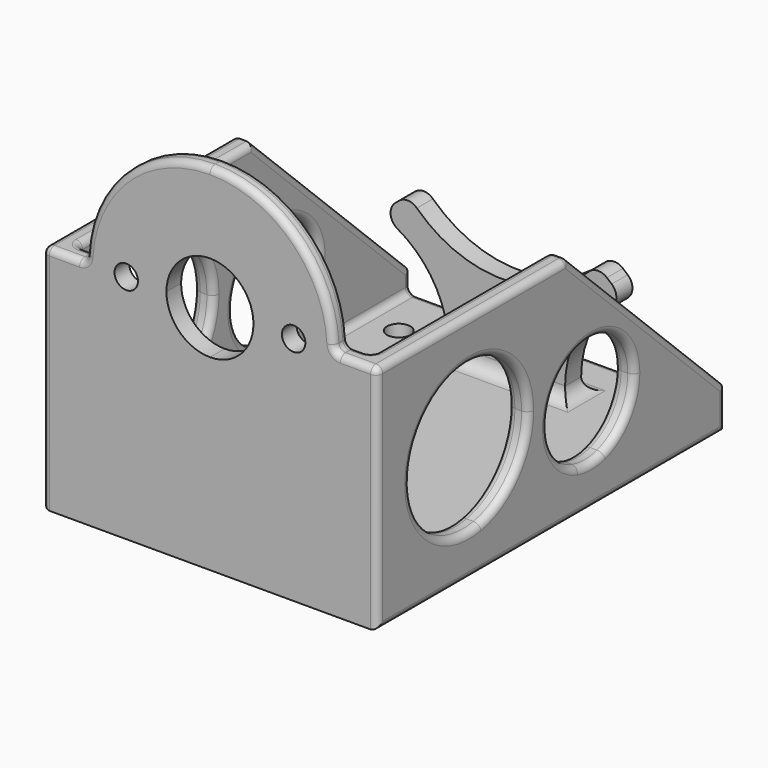
from build123d import *

# Parameters (mm, degrees)
F0_W      = 50
F0_H      = 65
F1_DEPTH  = 53
F2_W      = 44
F2_H      = 64
F3_DEPTH  = 50
F5_DEPTH  = 50.8
F6_R      = 1.75
F7_DEPTH  = 46.482
F9_DEPTH  = 51.054
F10_R     = 1
F12_DEPTH = 25.4
F14_DEPTH = 31.5
F16_DEPTH = 25.4
F17_R     = 2


with BuildPart() as f1:
    # F0 (on Top) → F1 (new body)
    with BuildSketch(Plane.XY):
        Rectangle(F0_W, F0_H)
    extrude(amount=F1_DEPTH)

    # F2 (on face) → F3 (cut)
    with BuildSketch(Plane.XY.offset(53)):
        with Locations((0, 2.2385166958)):
            Rectangle(F2_W, F2_H)
    extrude(amount=-F3_DEPTH, mode=Mode.SUBTRACT)

    # F4 (on face) → F5 (cut)
    with BuildSketch(Plane.YZ.offset(25)):
        Polygon((32.5, 53), (-16.1271169782, 53), (32.5, 6.0290149413), align=None)
    extrude(amount=-F5_DEPTH, mode=Mode.SUBTRACT)

    # F6 (on face) → F7 (cut)
    with BuildSketch(Plane.XZ.offset(32.5)):
        with Locations((-12.5, 34.5)):
            Circle(F6_R)
        with BuildLine():
            ThreePointArc((14.25, 34.5), (12.5, 36.25), (10.75, 34.5))
            ThreePointArc((10.75, 34.5), (12.5, 32.75), (14.25, 34.5))
        make_face()
        with BuildLine():
            Line((-6.5, 34.5), (0, 34.5))
            Line((0, 34.5), (6.5, 34.5))
            ThreePointArc((6.5, 34.5), (0, 41), (-6.5, 34.5))
        make_face()
        with BuildLine():
            Line((0, 34.5), (0, 28))
            ThreePointArc((0, 28), (4.5961940777, 29.9038059223), (6.5, 34.5))
            Line((6.5, 34.5), (0, 34.5))
        make_face()
        with BuildLine():
            ThreePointArc((-6.5, 34.5), (-4.5961940777, 29.9038059223), (0, 28))
            Line((0, 28), (0, 34.5))
            Line((0, 34.5), (-6.5, 34.5))
        make_face()
        with BuildLine():
            Line((-25, 34.5), (-18.5, 34.5))
            ThreePointArc((-18.5, 34.5), (-13.0814754005, 47.5814755034), (1.455e-07, 53))
            Line((1.455e-07, 53), (-25, 53))
            Line((-25, 53), (-25, 34.5))
        make_face()
        with BuildLine():
            Line((18.4999672276, 34.5348220845), (25, 34.5348220845))
            Line((25, 34.5348220845), (25, 53))
            Line((25, 53), (1.455e-07, 53))
            ThreePointArc((1.455e-07, 53), (13.0691582386, 47.5937810787), (18.4999672276, 34.5348220845))
        make_face()
    extrude(amount=-F7_DEPTH, mode=Mode.SUBTRACT)

    # F8 (on face) → F9 (cut)
    with BuildSketch(Plane.YZ.offset(25)):
        with BuildLine():
            ThreePointArc((-13.3143774193, 6.4202223538), (-6.8490219642, 10.2160643664), (-4.3019161944, 17.2674110422))
            ThreePointArc((-4.3019161944, 17.2674110422), (-23.8226956348, 24.3187577181), (-13.3143774193, 6.4202223538))
        make_face()
        with BuildLine():
            ThreePointArc((15.5232148034, 14.1681963578), (2.6051878457, 20.6598379602), (5.1052235569, 6.4202223538))
            Line((5.1052235569, 6.4202223538), (9.7609618177, 6.4202223538))
            ThreePointArc((9.7609618177, 6.4202223538), (13.9247342897, 9.3402915162), (15.5232148034, 14.1681963578))
        make_face()
        with BuildLine():
            Line((9.7609618177, 6.4202223538), (5.1052235569, 6.4202223538))
            ThreePointArc((5.1052235569, 6.4202223538), (7.4330926873, 6.0780742416), (9.7609618177, 6.4202223538))
        make_face()
    extrude(amount=-F9_DEPTH, mode=Mode.SUBTRACT)

    # F10
    f10_edges = [f1.edges().sort_by_distance(p)[0] for p in [
        (25, 0, 0),
        (25, -32.5, 17.267411),
        (25, 32.5, 3.014507),
        (25, -14.755441, 34.534822),
        (25, 17.744559, 20.281919),
        (25, -26.369801, 17.267411),
        (25, 9.760962, 21.91617),
        (-22, -13.368158, 34.5),
        (-22, 17.762584, 20.264507),
        (-22, -29.761483, 18.75),
        (-22, 32.5, 4.514507),
        (-22, 1.369258, 3),
        (-22, 9.760962, 21.91617),
        (-22, -26.369801, 17.267411),
        (22, -13.386183, 34.534822),
        (22, -29.761483, 18.767411),
        (22, 17.744559, 20.281919),
        (22, 1.369258, 3),
        (22, 32.5, 4.514507),
        (22, 9.760962, 21.91617),
        (22, -26.369801, 17.267411),
        (-25, 0, 0),
        (-25, 32.5, 3.014507),
        (-25, -32.5, 17.25),
        (-25, 17.762584, 20.264507),
        (-25, -14.737416, 34.5),
        (-25, -26.369801, 17.267411),
        (-25, 9.760962, 21.91617),
        (0, 32.5, 3),
        (0, -29.761483, 3),
        (-0.017411, -29.761483, 52.999992),
        (21.749984, -32.5, 34.534822),
        (23.5, 2.989118, 34.534822),
        (20.249984, -29.761483, 34.534822),
        (18.499967, -31.130742, 34.534822),
        (-21.75, -32.5, 34.5),
        (-0.017411, -32.5, 52.999992),
        (-18.5, -31.130742, 34.5),
        (-20.25, -29.761483, 34.5),
    ]]
    fillet(f10_edges, radius=F10_R)

    # F11 (on face) → F12 (cut)
    with BuildSketch(Plane.XY.offset(3)):
        with BuildLine():
            ThreePointArc((-15.25, 24), (-18.2374368671, 25.2374368671), (-17, 22.25))
            Line((-17, 22.25), (-17, 24))
            Line((-17, 24), (-15.25, 24))
        make_face()
        with BuildLine():
            Line((17, 24), (17, 22.25))
            ThreePointArc((17, 22.25), (18.2374368671, 22.7625631329), (18.75, 24))
            ThreePointArc((18.75, 24), (17, 25.75), (15.25, 24))
            Line((15.25, 24), (17, 24))
        make_face()
        with BuildLine():
            ThreePointArc((15.25, 24), (15.7625631329, 22.7625631329), (17, 22.25))
            Line((17, 22.25), (17, 24))
            Line((17, 24), (15.25, 24))
        make_face()
        with BuildLine():
            Line((-17, 24), (-17, 22.25))
            ThreePointArc((-17, 22.25), (-15.7625631329, 22.7625631329), (-15.25, 24))
            Line((-15.25, 24), (-17, 24))
        make_face()
        with BuildLine():
            Line((17, -24), (15.25, -24))
            ThreePointArc((15.25, -24), (17, -25.75), (18.75, -24))
            ThreePointArc((18.75, -24), (18.2374368671, -22.7625631329), (17, -22.25))
            Line((17, -22.25), (17, -24))
        make_face()
        with BuildLine():
            Line((-15.25, -24), (-17, -24))
            Line((-17, -24), (-17, -22.25))
            ThreePointArc((-17, -22.25), (-18.2374368671, -25.2374368671), (-15.25, -24))
        make_face()
        with BuildLine():
            ThreePointArc((17, -22.25), (15.7625631329, -22.7625631329), (15.25, -24))
            Line((15.25, -24), (17, -24))
            Line((17, -24), (17, -22.25))
        make_face()
        with BuildLine():
            Line((-17, -22.25), (-17, -24))
            Line((-17, -24), (-15.25, -24))
            ThreePointArc((-15.25, -24), (-15.7625631329, -22.7625631329), (-17, -22.25))
        make_face()
    extrude(amount=-F12_DEPTH, mode=Mode.SUBTRACT)

    # F13 (on face) → F14 (join)
    with BuildSketch(Plane.XY.offset(3)):
        Polygon((-18.5, 25.1999522895), (-18.5, 22.1999522895), (0, 22.1999522895), (18.5, 22.1999522895), (18.5, 25.1999522895), align=None)
    extrude(amount=F14_DEPTH)

    # F15 (on face) → F16 (cut)
    with BuildSketch(Plane(origin=(0, 25.1999522895, 0), x_dir=(-1, 0, 0), z_dir=(0, 1, 0))):
        with BuildLine():
            ThreePointArc((14.0864794815, 22.5074566577), (17.3615936827, 28.1105505091), (18.5, 34.5))
            Line((18.5, 34.5), (0, 34.5))
            Line((0, 34.5), (14.0864794815, 22.5074566577))
        make_face()
        with BuildLine():
            Line((0, 34.5), (-18.5, 34.5))
            ThreePointArc((-18.5, 34.5), (-17.3615936827, 28.1105505091), (-14.0864794815, 22.5074566577))
            Line((-14.0864794815, 22.5074566577), (0, 34.5))
        make_face()
        with BuildLine():
            ThreePointArc((-9.4374958426, 3), (-11.266359198, 12.4299466057), (-18.5, 18.75))
            Line((-18.5, 18.75), (-18.5, 3))
            Line((-18.5, 3), (-18.2738188659, 3))
            Line((-18.2738188659, 3), (-15.7261811341, 3))
            Line((-15.7261811341, 3), (-9.4374958426, 3))
        make_face()
        with BuildLine():
            Line((18.5, 3), (18.5, 18.75))
            ThreePointArc((18.5, 18.75), (10.5776127679, 12.6871084903), (8.1937499344, 3))
            Line((8.1937499344, 3), (15.7261811341, 3))
            Line((15.7261811341, 3), (18.2738188659, 3))
            Line((18.2738188659, 3), (18.5, 3))
        make_face()
        with BuildLine():
            ThreePointArc((-14.0864794815, 22.5074566577), (0, 16), (14.0864794815, 22.5074566577))
            Line((14.0864794815, 22.5074566577), (0, 34.5))
            Line((0, 34.5), (-14.0864794815, 22.5074566577))
        make_face()
        with BuildLine():
            Line((18.5, 18.75), (18.5, 34.5))
            ThreePointArc((18.5, 34.5), (17.3615936827, 28.1105505091), (14.0864794815, 22.5074566577))
            Line((14.0864794815, 22.5074566577), (18.5, 18.75))
        make_face()
        with BuildLine():
            ThreePointArc((-14.0864794815, 22.5074566577), (-17.3615936827, 28.1105505091), (-18.5, 34.5))
            Line((-18.5, 34.5), (-18.5, 18.75))
            Line((-18.5, 18.75), (-14.0864794815, 22.5074566577))
        make_face()
    extrude(amount=-F16_DEPTH, mode=Mode.SUBTRACT)

    # F17
    f17_edges = [f1.edges().sort_by_distance(p)[0] for p in [
        (14.086479, 23.699952, 22.507457),
        (-14.086479, 23.699952, 22.507457),
        (9.437496, 23.699952, 3),
        (0.621873, 25.199952, 3),
        (-8.19375, 23.699952, 3),
        (0.621873, 22.199952, 3),
        (18.5, 23.699952, 18.75),
        (-18.5, 23.699952, 18.75),
    ]]
    fillet(f17_edges, radius=F17_R)


solid = f1.part
